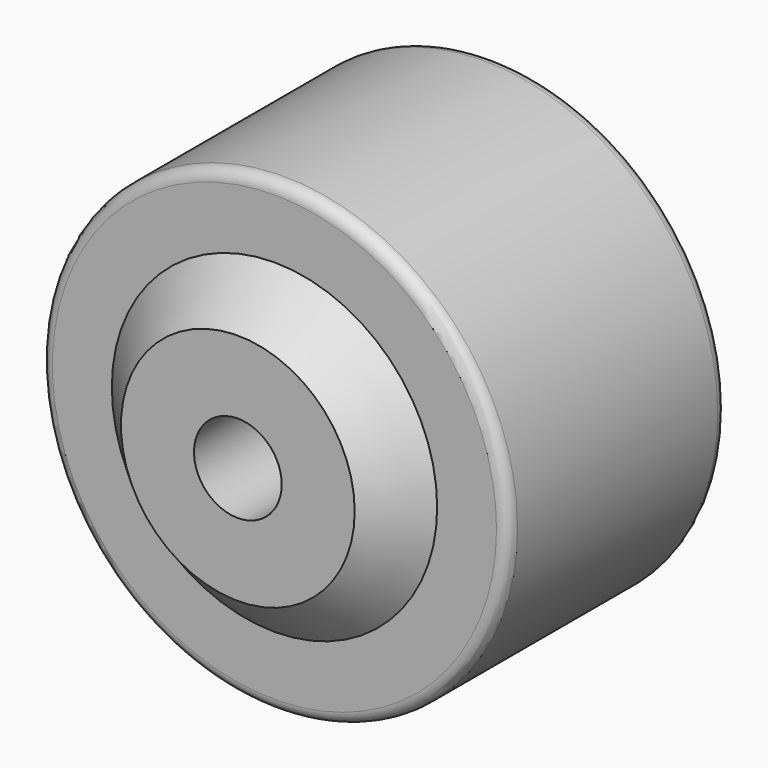
from build123d import *

# Parameters (mm, degrees)
F0_R     = 19.05
F0_R_2   = 4.7625
F1_DEPTH = 19.8374
F0_R_3   = 25.4
F2_DEPTH = 14.859
F4_R     = 1.27


# Not quite as in the source:
# - a fillet or chamfer that OpenCascade refuses, or shapes differently, is made with other operations: its cross-section is extruded or revolved along the edge and cut away or added


with BuildPart() as f1:
    # F0 (on Front) → F1 (new body, symmetric)
    with BuildSketch(Plane.XZ):
        Circle(F0_R)
        Circle(F0_R_2, mode=Mode.SUBTRACT)
    extrude(amount=F1_DEPTH, both=True)

    # F0 (on Front) → F2 (join, symmetric)
    with BuildSketch(Plane.XZ):
        Circle(F0_R_3)
        Circle(F0_R, mode=Mode.SUBTRACT)
    extrude(amount=F2_DEPTH, both=True)

    # F3: chamfer of 6.35 on 2 edges, made by hand


with BuildPart() as f3_tool2:
    # F3_s3 → F3_t4 (revolve)
    with BuildSketch(Plane.XY):
        Polygon((12.7, -19.8374), (19.05, -13.4874), (19.05, -19.8374), align=None)
    revolve(axis=Axis((0, -19.8374, 0), (0, -1, 0)))

    split(bisect_by=Plane.XZ.offset(14.859), keep=Keep.TOP)


with BuildPart() as f1_1:
    add(f1.part)

    # F3_t1: cut F3_tool2
    add(f3_tool2.part, mode=Mode.SUBTRACT)


with BuildPart() as f3_tool7:
    # F3_s8 → F3_t9 (revolve)
    with BuildSketch(Plane.XY):
        Polygon((19.05, 13.4874), (12.7, 19.8374), (19.05, 19.8374), align=None)
    revolve(axis=Axis((0, 19.8374, 0), (0, -1, 0)))

    split(bisect_by=Plane.XZ.offset(-14.859), keep=Keep.BOTTOM)


with BuildPart() as f1_2:
    add(f1_1.part)

    # F3_t6: cut F3_tool7
    add(f3_tool7.part, mode=Mode.SUBTRACT)

    # F4
    f4_edges = [f1_2.edges().sort_by_distance(p)[0] for p in [
        (-25.4, -14.859, 0),
        (-25.4, 14.859, 0),
    ]]
    fillet(f4_edges, radius=F4_R)


solid = f1_2.part
